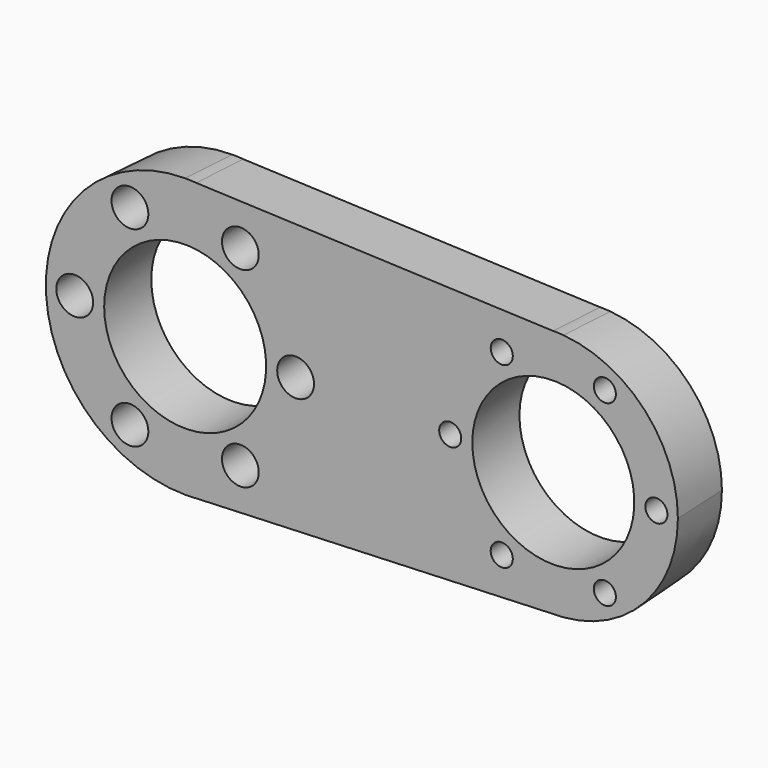
from build123d import *

# Parameters (mm, degrees)
F1_DEPTH = 8
F1_TAPER = -3
F3_D     = 22
F4_D     = 22
F6_D     = 5
F7_D     = 3


# Not quite as in the source:
# - a feature of the source that left no trace in its solid (it failed there, or was rolled back) is left out


with BuildPart() as f1:
    # F0 (on Front) → F1 (new body)
    with BuildSketch(Plane.XZ):
        with BuildLine():
            Line((1.4786393064, 18.4408141307), (0, 18.5))
            ThreePointArc((0, 18.5), (-18.5, 0), (0, -18.5))
            Line((0, -18.5), (1.4786393064, -18.4408141307))
            ThreePointArc((1.4786393064, -18.4408141307), (13.5942051472, -12.5478120171), (18.5, 0))
            ThreePointArc((18.5, 0), (13.5942051472, 12.5478120171), (1.4786393064, 18.4408141307))
        make_face()
        with BuildLine():
            ThreePointArc((1.4786393064, 18.4408141307), (0.7399116781, 18.4851976108), (0, 18.5))
            Line((0, 18.5), (1.4786393064, 18.4408141307))
        make_face()
        with BuildLine():
            Line((1.4786393064, -18.4408141307), (0, -18.5))
            ThreePointArc((0, -18.5), (0.7399116781, -18.4851976108), (1.4786393064, -18.4408141307))
        make_face()
        with BuildLine():
            Line((49.9667920397, 16.4999665827), (1.4786393064, 18.4408141307))
            ThreePointArc((1.4786393064, 18.4408141307), (13.5942051472, 12.5478120171), (18.5, 0))
            Line((18.5, 0), (33.5, 0))
            ThreePointArc((33.5, 0), (38.3210032249, 11.6555151893), (49.9667920397, 16.4999665827))
        make_face()
        with BuildLine():
            ThreePointArc((18.5, 0), (13.5942051472, -12.5478120171), (1.4786393064, -18.4408141307))
            Line((1.4786393064, -18.4408141307), (49.9667920397, -16.4999665827))
            ThreePointArc((49.9667920397, -16.4999665827), (38.3210032249, -11.6555151893), (33.5, 0))
            Line((33.5, 0), (18.5, 0))
        make_face()
        with BuildLine():
            Line((51.3518854576, 16.4445250983), (49.9667920397, 16.4999665827))
            ThreePointArc((49.9667920397, 16.4999665827), (38.3210032249, 11.6555151893), (33.5, 0))
            ThreePointArc((33.5, 0), (38.3210032249, -11.6555151893), (49.9667920397, -16.4999665827))
            Line((49.9667920397, -16.4999665827), (51.3518854576, -16.4445250983))
            ThreePointArc((51.3518854576, -16.4445250983), (62.1358170316, -11.1790851582), (66.5, 0))
            ThreePointArc((66.5, 0), (62.1358170316, 11.1790851582), (51.3518854576, 16.4445250983))
        make_face()
        with BuildLine():
            ThreePointArc((51.3518854576, 16.4445250983), (50.6599212264, 16.4867978691), (49.9667920397, 16.4999665827))
            Line((49.9667920397, 16.4999665827), (51.3518854576, 16.4445250983))
        make_face()
        with BuildLine():
            Line((51.3518854576, -16.4445250983), (49.9667920397, -16.4999665827))
            ThreePointArc((49.9667920397, -16.4999665827), (50.6599212264, -16.4867978691), (51.3518854576, -16.4445250983))
        make_face()
    extrude(amount=F1_DEPTH, taper=F1_TAPER)

    # F3 (through all)
    with Locations(Plane(origin=(0, 0, 0), x_dir=(1, 0, 0), z_dir=(0, 1, 0))):
        with Locations((50, 0)):
            Hole(F3_D / 2)

    # F4 (through all)
    with Locations(Plane(origin=(0, 0, 0), x_dir=(1, 0, 0), z_dir=(0, 1, 0))):
        with Locations((0, 0)):
            Hole(F4_D / 2)

    # F6 (through all)
    with Locations(Plane.XZ.offset(8)):
        with Locations((15, 0), (7.5, 12.9903810568), (-7.5, 12.9903810568), (-15, 0), (-7.5, -12.9903810568), (7.5, -12.9903810568)):
            Hole(F6_D / 2)

    # F7 (through all)
    with Locations(Plane.XZ.offset(8)):
        with Locations((36, 0), (43, 12.124355653), (57, 12.124355653), (64, 0), (57, -12.124355653), (43, -12.124355653)):
            Hole(F7_D / 2)


solid = f1.part
